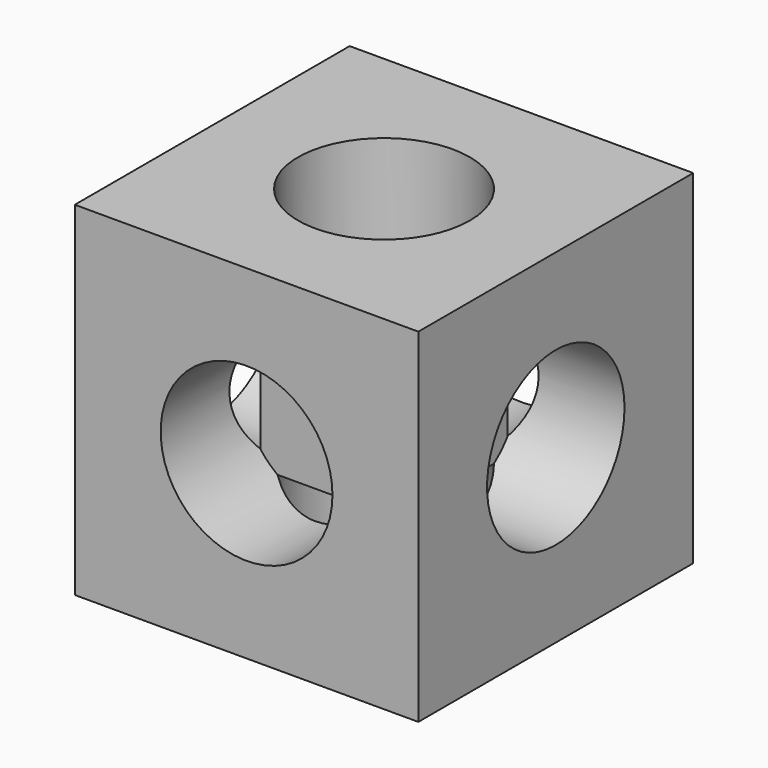
from build123d import *

# Parameters (mm, degrees)
F0_W      = 25.4
F0_H      = 25.4
F1_DEPTH  = 25.4
F2_R      = 6.35
F3_DEPTH  = 7.62
F4_R      = 6.35
F5_DEPTH  = 7.62
F6_R      = 6.35
F7_DEPTH  = 7.62
F8_R      = 6.35
F9_DEPTH  = 7.62
F10_R     = 6.35
F11_DEPTH = 7.62
F12_R     = 6.35
F13_DEPTH = 7.62


# Not quite as in the source:
# - a feature names something its author has since deleted; it is built from what else it names


with BuildPart() as f1:
    # F0 (on Front) → F1 (new body)
    with BuildSketch(Plane.XZ):
        Rectangle(F0_W, F0_H)
    extrude(amount=F1_DEPTH)

    # F2 (on face) → F3 (cut)
    with BuildSketch(Plane.XZ.offset(25.4)):
        Circle(F2_R)
    extrude(amount=-F3_DEPTH, mode=Mode.SUBTRACT)

    # F4 (on face) → F5 (cut)
    with BuildSketch(Plane(origin=(0, 0, 0), x_dir=(-1, 0, 0), z_dir=(0, 1, 0))):
        Circle(F4_R)
    extrude(amount=-F5_DEPTH, mode=Mode.SUBTRACT)

    # F6 (on face) → F7 (cut)
    with BuildSketch(Plane.YZ.offset(12.7)):
        with Locations((-12.7, 0)):
            Circle(F6_R)
    extrude(amount=-F7_DEPTH, mode=Mode.SUBTRACT)

    # F8 (on face) → F9 (cut)
    with BuildSketch(Plane(origin=(-12.7, 0, 0), x_dir=(0, -1, 0), z_dir=(-1, 0, 0))):
        with Locations((12.7, 0)):
            Circle(F8_R)
    extrude(amount=-F9_DEPTH, mode=Mode.SUBTRACT)

    # F10 (on face) → F11 (cut)
    with BuildSketch(Plane.XY.offset(12.7)):
        with Locations((0, -12.7)):
            Circle(F10_R)
    extrude(amount=-F11_DEPTH, mode=Mode.SUBTRACT)

    # F12 (on face) → F13 (cut)
    with BuildSketch(Plane(origin=(0, 0, -12.7), x_dir=(1, 0, 0), z_dir=(0, 0, -1))):
        with Locations((0, 12.7)):
            Circle(F12_R)
    extrude(amount=-F13_DEPTH, mode=Mode.SUBTRACT)


solid = f1.part
